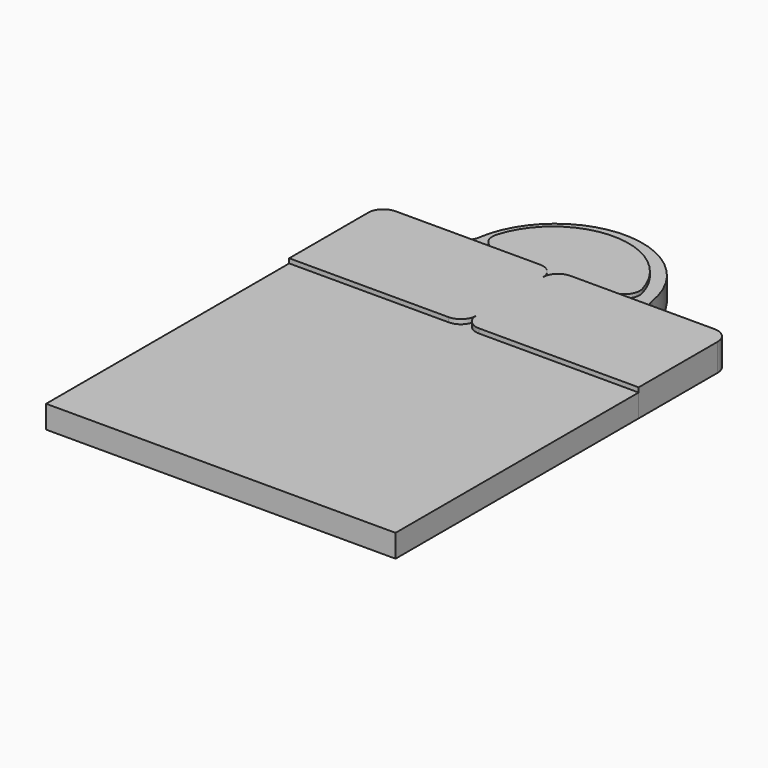
from build123d import *

# Parameters (mm, degrees)
F0_W     = 42.0281105638
F0_H     = 33.6269846465
F1_DEPTH = 3
F2_DEPTH = 3.6
F3_DEPTH = 3.5


# Not quite as in the source:
# - the program builds the solid bodies; features that only make, move or delete a surface that nothing else refers to are left out


with BuildPart() as f1:
    # F0 (on Top) → F1 (new body)
    with BuildSketch(Plane.XY):
        with BuildLine():
            Line((0, 40), (0, 0))
            Line((0, 0), (46, 0))
            Line((46, 0), (46, 40))
            Line((46, 40), (43, 40))
            Line((43, 40), (25, 40))
            ThreePointArc((25, 40), (23.5857864376, 40.5857864376), (23, 42))
            ThreePointArc((23, 42), (22.4142135624, 40.5857864376), (21, 40))
            Line((21, 40), (3, 40))
            Line((3, 40), (0, 40))
        make_face()
        with Locations((23, 19.8172420869)):
            Rectangle(F0_W, F0_H, mode=Mode.SUBTRACT)
        with Locations((23, 19.8172420869)):
            Rectangle(F0_W, F0_H)
    extrude(amount=F1_DEPTH)


with BuildPart() as f1b:
    # F0 (on Top) → F1, piece 2 (new body)
    with BuildSketch(Plane.XY):
        with BuildLine():
            ThreePointArc((13.2436284078, 57.5546079039), (13.5668788118, 55.7977553926), (15.1651928936, 55))
            Line((15.1651928936, 55), (21, 55))
            ThreePointArc((21, 55), (22.4142135624, 54.4142135624), (23, 53))
            ThreePointArc((23, 53), (23.5857864376, 54.4142135624), (25, 55))
            Line((25, 55), (30.5447365354, 55))
            ThreePointArc((30.5447365354, 55), (32.1430506172, 55.7977553926), (32.4663010212, 57.5546079039))
            ThreePointArc((32.4663010212, 57.5546079039), (22.8549647145, 64.7842115073), (13.2436284078, 57.5546079039))
        make_face()
        with BuildLine():
            ThreePointArc((11.6269004361, 56.7037037037), (10.954230091, 55.4846464781), (9.6489700772, 55))
            Line((9.6489700772, 55), (15.1651928936, 55))
            ThreePointArc((15.1651928936, 55), (13.5668788118, 55.7977553926), (13.2436284078, 57.5546079039))
            ThreePointArc((13.2436284078, 57.5546079039), (22.8549647145, 64.7842115073), (32.4663010212, 57.5546079039))
            ThreePointArc((32.4663010212, 57.5546079039), (32.1430506172, 55.7977553926), (30.5447365354, 55))
            Line((30.5447365354, 55), (36.3510299228, 55))
            ThreePointArc((36.3510299228, 55), (35.045769909, 55.4846464781), (34.3730995639, 56.7037037037))
            ThreePointArc((34.3730995639, 56.7037037037), (23, 66.5), (11.6269004361, 56.7037037037))
        make_face()
    extrude(amount=F1_DEPTH)


with BuildPart() as f2:
    # F0 (on Top) → F2 (new body)
    with BuildSketch(Plane.XY):
        with BuildLine():
            Line((0, 53), (0, 40))
            Line((0, 40), (3, 40))
            Line((3, 40), (21, 40))
            ThreePointArc((21, 40), (22.4142135624, 40.5857864376), (23, 42))
            Line((23, 42), (23, 53))
            ThreePointArc((23, 53), (22.4142135624, 54.4142135624), (21, 55))
            Line((21, 55), (15.1651928936, 55))
            Line((15.1651928936, 55), (9.6489700772, 55))
            Line((9.6489700772, 55), (2, 55))
            ThreePointArc((2, 55), (0.5857864376, 54.4142135624), (0, 53))
        make_face()
        with BuildLine():
            Line((43, 40), (46, 40))
            Line((46, 40), (46, 53))
            ThreePointArc((46, 53), (45.4142135624, 54.4142135624), (44, 55))
            Line((44, 55), (36.3510299228, 55))
            Line((36.3510299228, 55), (30.5447365354, 55))
            Line((30.5447365354, 55), (25, 55))
            ThreePointArc((25, 55), (23.5857864376, 54.4142135624), (23, 53))
            Line((23, 53), (23, 42))
            ThreePointArc((23, 42), (23.5857864376, 40.5857864376), (25, 40))
            Line((25, 40), (43, 40))
        make_face()
    extrude(amount=F2_DEPTH)


with BuildPart() as f3:
    # F0 (on Top) → F3 (new body)
    with BuildSketch(Plane.XY):
        with BuildLine():
            ThreePointArc((13.2436284078, 57.5546079039), (13.5668788118, 55.7977553926), (15.1651928936, 55))
            Line((15.1651928936, 55), (21, 55))
            ThreePointArc((21, 55), (22.4142135624, 54.4142135624), (23, 53))
            ThreePointArc((23, 53), (23.5857864376, 54.4142135624), (25, 55))
            Line((25, 55), (30.5447365354, 55))
            ThreePointArc((30.5447365354, 55), (32.1430506172, 55.7977553926), (32.4663010212, 57.5546079039))
            ThreePointArc((32.4663010212, 57.5546079039), (22.8549647145, 64.7842115073), (13.2436284078, 57.5546079039))
        make_face()
    extrude(amount=F3_DEPTH)


solid = Compound([f1.part, f1b.part, f2.part, f3.part])
